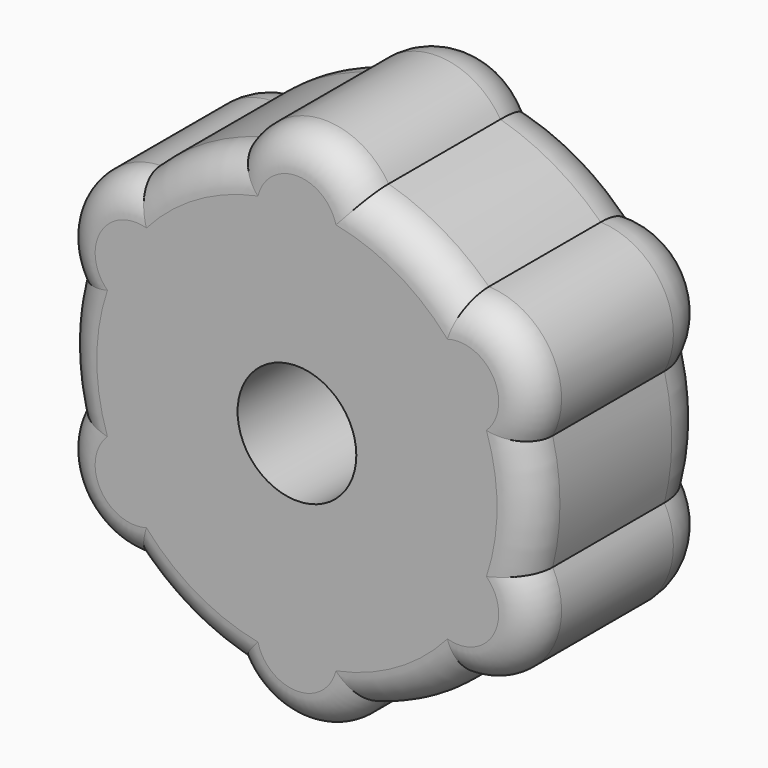
from build123d import *

# Parameters (mm, degrees)
F0_R         = 6.477
F1_DEPTH     = 25.4
F2_R         = 3.81
F3_R         = 6.35
F4_TEXT_SIZE = 11.1006523689
F5_DEPTH     = 0.762


# Not quite as in the source:
# - Text() gives the source's letters only with a copy of the font that has no kerning and outlines rounded to 1/6400 em; it was checked with that copy


with BuildPart() as f1:
    # F0 (on Front) → F1 (new body)
    with BuildSketch(Plane.XZ):
        with BuildLine():
            ThreePointArc((6.9580851201, 24.6804503002), (0, 28.5475678146), (-6.9580851201, 24.6804503002))
            ThreePointArc((-6.9580851201, 24.6804503002), (-12.8212672498, 22.207086294), (-17.8948543768, 18.3661036258))
            ThreePointArc((-17.8948543768, 18.3661036258), (-24.7229189437, 14.2737839073), (-24.8529394969, 6.3143466744))
            ThreePointArc((-24.8529394969, 6.3143466744), (-25.6425344996, 0), (-24.8529394969, -6.3143466744))
            ThreePointArc((-24.8529394969, -6.3143466744), (-24.7229189437, -14.2737839073), (-17.8948543768, -18.3661036258))
            ThreePointArc((-17.8948543768, -18.3661036258), (-12.8212672498, -22.207086294), (-6.9580851201, -24.6804503002))
            ThreePointArc((-6.9580851201, -24.6804503002), (0, -28.5475678146), (6.9580851201, -24.6804503002))
            ThreePointArc((6.9580851201, -24.6804503002), (12.8212672498, -22.207086294), (17.8948543768, -18.3661036258))
            ThreePointArc((17.8948543768, -18.3661036258), (24.7229189437, -14.2737839073), (24.8529394969, -6.3143466744))
            ThreePointArc((24.8529394969, -6.3143466744), (25.6425344996, 0), (24.8529394969, 6.3143466744))
            ThreePointArc((24.8529394969, 6.3143466744), (24.7229189437, 14.2737839073), (17.8948543768, 18.3661036258))
            ThreePointArc((17.8948543768, 18.3661036258), (12.8212672498, 22.207086294), (6.9580851201, 24.6804503002))
        make_face()
        Circle(F0_R, mode=Mode.SUBTRACT)
    extrude(amount=F1_DEPTH)

    # F2
    f2_edges = [f1.edges().sort_by_distance(p)[0] for p in [
        (-25.642534, -25.4, 0),
        (-24.722919, -25.4, -14.273784),
        (-12.821267, -25.4, -22.207086),
        (-24.722919, -25.4, 14.273784),
        (-12.821267, -25.4, 22.207086),
        (0, -25.4, 28.547568),
        (12.821267, -25.4, 22.207086),
        (24.722919, -25.4, 14.273784),
        (25.642534, -25.4, 0),
        (24.722919, -25.4, -14.273784),
        (12.821267, -25.4, -22.207086),
        (0, -25.4, -28.547568),
    ]]
    fillet(f2_edges, radius=F2_R)

    # F3
    f3_edges = [f1.edges().sort_by_distance(p)[0] for p in [
        (-12.821267, 0, 22.207086),
        (0, 0, 28.547568),
        (12.821267, 0, 22.207086),
        (24.722919, 0, 14.273784),
        (25.642534, 0, 0),
        (24.722919, 0, -14.273784),
        (12.821267, 0, -22.207086),
        (0, 0, -28.547568),
        (-12.821267, 0, -22.207086),
        (-24.722919, 0, -14.273784),
        (-25.642534, 0, 0),
        (-24.722919, 0, 14.273784),
    ]]
    fillet(f3_edges, radius=F3_R)

    # F4 (on face) → F5 (join)
    with BuildSketch(Plane(origin=(0, 0, 0), x_dir=(-1, 0, 0), z_dir=(0, 1, 0))):
        with Locations((-9.5281116664, 9.065956343)):
            Text('MJL', F4_TEXT_SIZE, font='Open Sans', font_style=FontStyle.BOLD, text_align=(TextAlign.LEFT, TextAlign.BOTTOM))
    extrude(amount=F5_DEPTH)


solid = f1.part
